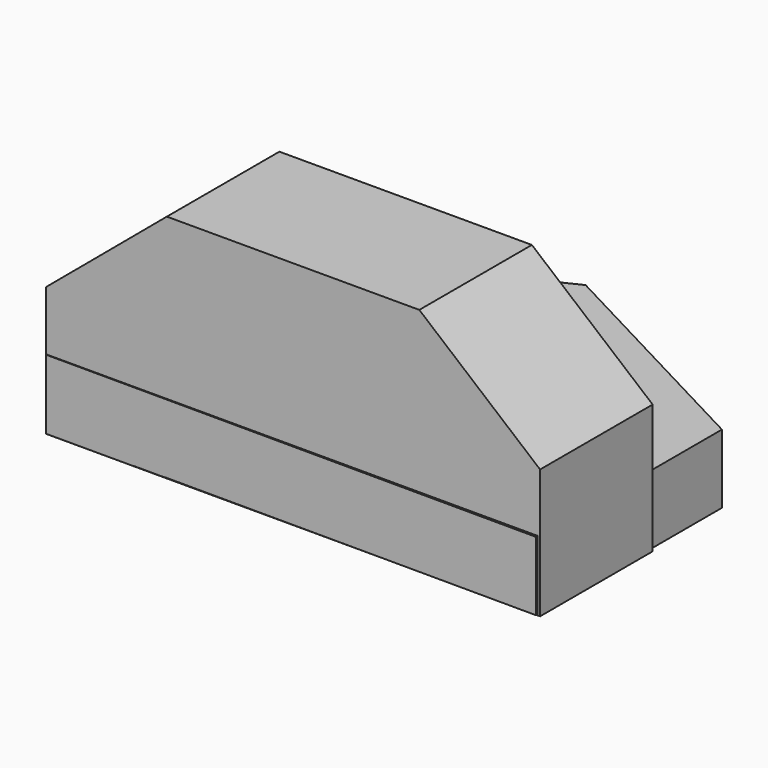
from build123d import *

# Parameters (mm, degrees)
F1_DEPTH    = 25.4
F3_DEPTH    = 12.446
F4_W        = 11.3675398752
F4_H        = 8.0155739561
F4_W_2      = 11.0760703683
F4_H_2      = 7.7240983956
F5_DEPTH    = 14.224
F6_T4_DEPTH = 76.6882877695
F7_T4_DEPTH = 76.3968182626


# Not quite as in the source:
# - a fillet or chamfer that OpenCascade refuses, or shapes differently, is made with other operations: its cross-section is extruded or revolved along the edge and cut away or added


with BuildPart() as f1:
    # F0 (on Front) → F1 (new body)
    with BuildSketch(Plane.XZ):
        Polygon((-56.9788375091, 10.6936474436), (-56.9788375091, -12.6478849719), (32.2034358534, -12.6478849719), (32.2034358534, 10.6936474436), (10.4033187203, 28.9705070476), (-35.1787281407, 28.9705070476), align=None)
    extrude(amount=F1_DEPTH)

    # F2 (on Top) → F3 (join)
    with BuildSketch(Plane.XY):
        Polygon((-56.8377040327, 0), (-56.8377040327, -25.5040973425), (31.7708179355, -25.7955752313), (31.7708179355, 0), align=None)
        Polygon((-56.8377040327, 16.1768849939), (-56.8377040327, 0), (31.7708179355, 0), (31.7708179355, 16.1768849939), (-10.7845906168, 38.6204943061), align=None)
    extrude(amount=-F3_DEPTH)

    # F4 (on Front) → F5 (join)
    with BuildSketch(Plane.XZ):
        with Locations((13.5536068119, 4.007786978)):
            Rectangle(F4_W, F4_H)
        with Locations((-31.1878696084, 3.8620491978)):
            Rectangle(F4_W_2, F4_H_2)
    extrude(amount=-F5_DEPTH)

    # F6: chamfer of 12.7 on 1 edges, made by hand


with BuildPart() as f6_tool2:
    # F6_s3 → F6_t4 (new body)
    with BuildSketch(Plane.YZ.offset(51.8977506967)):
        Polygon((1.524, 8.0155739561), (14.224, -4.6844260439), (14.224, 8.0155739561), align=None)
    extrude(amount=-F6_T4_DEPTH)

    split(bisect_by=Plane.XY, keep=Keep.TOP)


with BuildPart() as f1_1:
    add(f1.part)

    # F6_t1: cut F6_tool2
    add(f6_tool2.part, mode=Mode.SUBTRACT)

    # F7: chamfer of 12.7 on 1 edges, made by hand


with BuildPart() as f7_tool2:
    # F7_s3 → F7_t4 (new body)
    with BuildSketch(Plane.YZ.offset(7.0105395229)):
        Polygon((14.224, -4.9759016044), (1.524, 7.7240983956), (14.224, 7.7240983956), align=None)
    extrude(amount=-F7_T4_DEPTH)

    split(bisect_by=Plane.XY, keep=Keep.TOP)


with BuildPart() as f1_2:
    add(f1_1.part)

    # F7_t1: cut F7_tool2
    add(f7_tool2.part, mode=Mode.SUBTRACT)


solid = f1_2.part
